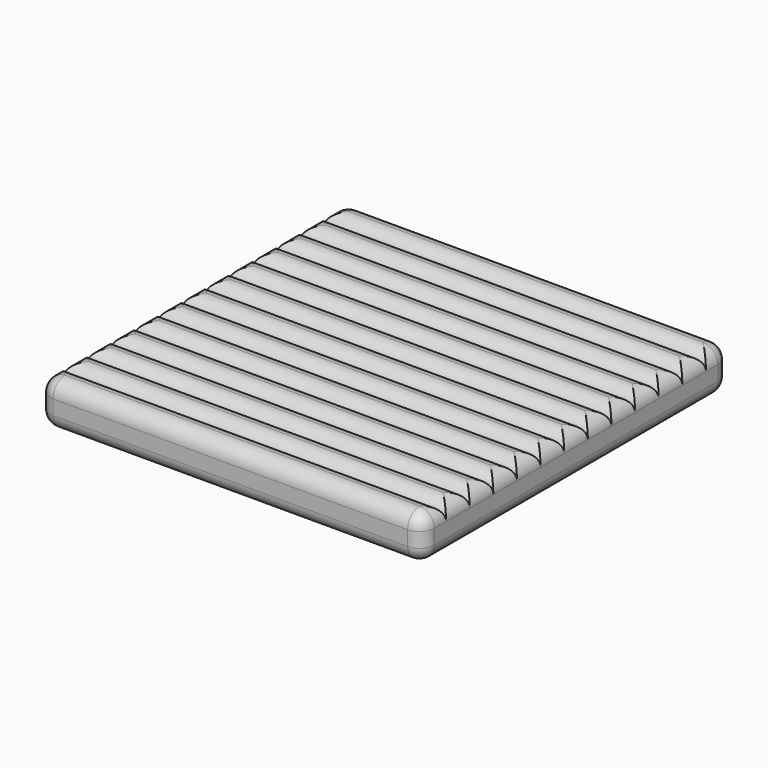
from build123d import *

# Parameters (mm, degrees)
F0_W         = 330.2
F0_H         = 330.2
F1_DEPTH     = 38.1
F2_R         = 12.7
F3_T1_DEPTH  = 12.7
F3_S5_W      = 12.7
F3_S5_H      = 12.7
F3_T6_DEPTH  = 12.7
F3_S11_W     = 12.7
F3_S11_H     = 12.7
F3_T12_DEPTH = 12.7
F3_S17_W     = 12.7
F3_S17_H     = 12.7
F3_T18_DEPTH = 12.7
F3_S23_W     = 12.7
F3_S23_H     = 12.7
F3_T24_DEPTH = 12.7
F3_S29_W     = 12.7
F3_S29_H     = 12.7
F3_T30_DEPTH = 12.7
F3_S35_W     = 12.7
F3_S35_H     = 12.7
F3_T36_DEPTH = 12.7
F3_S41_W     = 12.7
F3_S41_H     = 12.7
F3_T42_DEPTH = 12.7
F3_S47_W     = 12.7
F3_S47_H     = 12.7
F3_T48_DEPTH = 12.7
F5_DEPTH     = 330.201


# Not quite as in the source:
# - a fillet or chamfer that OpenCascade refuses, or shapes differently, is made with other operations: its cross-section is extruded or revolved along the edge and cut away or added
# - ends of sketch curves that miss each other by under 0.0002 mm in the source are joined


with BuildPart() as f1:
    # F0 (on Top) → F1 (new body)
    with BuildSketch(Plane.XY):
        with Locations((165.1, 165.1)):
            Rectangle(F0_W, F0_H)
    extrude(amount=F1_DEPTH)

    # F2
    f2_edges = [f1.edges().sort_by_distance(p)[0] for p in [
        (0, 165.1, 38.1),
        (165.1, 0, 38.1),
        (330.2, 165.1, 38.1),
        (165.1, 330.2, 38.1),
        (0, 165.1, 0),
        (165.1, 0, 0),
        (330.2, 165.1, 0),
        (165.1, 330.2, 0),
    ]]
    fillet(f2_edges, radius=F2_R)

    # F3: fillet of radius 12.7 on 4 edges, made by hand

    # F3_s2 → F3_t1 (cut)
    with BuildSketch(Plane.XY.offset(12.7)):
        with BuildLine():
            ThreePointArc((0, 12.7), (3.7197438789, 3.7197438789), (12.7, 0))
            Line((12.7, 0), (0, 0))
            Line((0, 0), (0, 12.7))
        make_face()
        with BuildLine():
            ThreePointArc((0, 317.5), (3.7197438789, 326.4802561211), (12.7, 330.2))
            Line((12.7, 330.2), (0, 330.2))
            Line((0, 330.2), (0, 317.5))
        make_face()
        with BuildLine():
            ThreePointArc((317.5, 330.2), (326.4802561211, 326.4802561211), (330.2, 317.5))
            Line((330.2, 317.5), (330.2, 330.2))
            Line((330.2, 330.2), (317.5, 330.2))
        make_face()
        with BuildLine():
            ThreePointArc((317.5, 0), (326.4802561211, 3.7197438789), (330.2, 12.7))
            Line((330.2, 12.7), (330.2, 0))
            Line((330.2, 0), (317.5, 0))
        make_face()
    extrude(amount=F3_T1_DEPTH, mode=Mode.SUBTRACT)


with BuildPart() as f3_tool4:
    # F3_s5 → F3_t6 (new body)
    with BuildSketch(Plane.XZ.offset(-12.7)):
        with Locations((323.85, 6.35)):
            Rectangle(F3_S5_W, F3_S5_H)
    extrude(amount=F3_T6_DEPTH)

    # F3_s7 → F3_t8 (revolve, cut)
    with BuildSketch(Plane(origin=(317.5, 12.7, 12.7), x_dir=(-0.7071067812, 0, 0.7071067812), z_dir=(0.7071067812, 0, 0.7071067812))):
        with BuildLine():
            ThreePointArc((0, -12.7), (12.7, 0), (0, 12.7))
            Line((0, 12.7), (0, -12.7))
        make_face()
    revolve(axis=Axis((317.5, 12.7, 12.7), (0, -1, 0)), mode=Mode.SUBTRACT)


with BuildPart() as f1_1:
    add(f1.part)

    # F3_t3: cut F3_tool4
    add(f3_tool4.part, mode=Mode.SUBTRACT)


with BuildPart() as f3_tool10:
    # F3_s11 → F3_t12 (new body)
    with BuildSketch(Plane.XZ.offset(-12.7)):
        with Locations((323.85, 31.75)):
            Rectangle(F3_S11_W, F3_S11_H)
    extrude(amount=F3_T12_DEPTH)

    # F3_s13 → F3_t14 (revolve, cut)
    with BuildSketch(Plane(origin=(317.5, 12.7, 25.4), x_dir=(-0.7071067812, 0, -0.7071067812), z_dir=(-0.7071067812, 0, 0.7071067812))):
        with BuildLine():
            ThreePointArc((0, -12.7), (12.7, 0), (0, 12.7))
            Line((0, 12.7), (0, -12.7))
        make_face()
    revolve(axis=Axis((317.5, 12.7, 25.4), (0, -1, 0)), mode=Mode.SUBTRACT)


with BuildPart() as f1_2:
    add(f1_1.part)

    # F3_t9: cut F3_tool10
    add(f3_tool10.part, mode=Mode.SUBTRACT)


with BuildPart() as f3_tool16:
    # F3_s17 → F3_t18 (new body)
    with BuildSketch(Plane.XZ.offset(-317.5)):
        with Locations((323.85, 6.35)):
            Rectangle(F3_S17_W, F3_S17_H)
    extrude(amount=-F3_T18_DEPTH)

    # F3_s19 → F3_t20 (revolve, cut)
    with BuildSketch(Plane(origin=(317.5, 317.5, 12.7), x_dir=(-0.7071067812, 0, 0.7071067812), z_dir=(-0.7071067812, 0, -0.7071067812))):
        with BuildLine():
            ThreePointArc((0, -12.7), (12.7, 0), (0, 12.7))
            Line((0, 12.7), (0, -12.7))
        make_face()
    revolve(axis=Axis((317.5, 317.5, 12.7), (0, 1, 0)), mode=Mode.SUBTRACT)


with BuildPart() as f1_3:
    add(f1_2.part)

    # F3_t15: cut F3_tool16
    add(f3_tool16.part, mode=Mode.SUBTRACT)


with BuildPart() as f3_tool22:
    # F3_s23 → F3_t24 (new body)
    with BuildSketch(Plane.XZ.offset(-317.5)):
        with Locations((323.85, 31.75)):
            Rectangle(F3_S23_W, F3_S23_H)
    extrude(amount=-F3_T24_DEPTH)

    # F3_s25 → F3_t26 (revolve, cut)
    with BuildSketch(Plane(origin=(317.5, 317.5, 25.4), x_dir=(-0.7071067812, 0, -0.7071067812), z_dir=(0.7071067812, 0, -0.7071067812))):
        with BuildLine():
            ThreePointArc((0, -12.7), (12.7, 0), (0, 12.7))
            Line((0, 12.7), (0, -12.7))
        make_face()
    revolve(axis=Axis((317.5, 317.5, 25.4), (0, 1, 0)), mode=Mode.SUBTRACT)


with BuildPart() as f1_4:
    add(f1_3.part)

    # F3_t21: cut F3_tool22
    add(f3_tool22.part, mode=Mode.SUBTRACT)


with BuildPart() as f3_tool28:
    # F3_s29 → F3_t30 (new body)
    with BuildSketch(Plane.YZ.offset(12.7)):
        with Locations((323.85, 6.35)):
            Rectangle(F3_S29_W, F3_S29_H)
    extrude(amount=-F3_T30_DEPTH)

    # F3_s31 → F3_t32 (revolve, cut)
    with BuildSketch(Plane(origin=(12.7, 317.5, 12.7), x_dir=(0, -0.7071067812, 0.7071067812), z_dir=(0, -0.7071067812, -0.7071067812))):
        with BuildLine():
            ThreePointArc((0, -12.7), (12.7, 0), (0, 12.7))
            Line((0, 12.7), (0, -12.7))
        make_face()
    revolve(axis=Axis((12.7, 317.5, 12.7), (-1, 0, 0)), mode=Mode.SUBTRACT)


with BuildPart() as f1_5:
    add(f1_4.part)

    # F3_t27: cut F3_tool28
    add(f3_tool28.part, mode=Mode.SUBTRACT)


with BuildPart() as f3_tool34:
    # F3_s35 → F3_t36 (new body)
    with BuildSketch(Plane.YZ.offset(12.7)):
        with Locations((323.85, 31.75)):
            Rectangle(F3_S35_W, F3_S35_H)
    extrude(amount=-F3_T36_DEPTH)

    # F3_s37 → F3_t38 (revolve, cut)
    with BuildSketch(Plane(origin=(12.7, 317.5, 25.4), x_dir=(0, -0.7071067812, -0.7071067812), z_dir=(0, 0.7071067812, -0.7071067812))):
        with BuildLine():
            ThreePointArc((0, -12.7), (12.7, 0), (0, 12.7))
            Line((0, 12.7), (0, -12.7))
        make_face()
    revolve(axis=Axis((12.7, 317.5, 25.4), (-1, 0, 0)), mode=Mode.SUBTRACT)


with BuildPart() as f1_6:
    add(f1_5.part)

    # F3_t33: cut F3_tool34
    add(f3_tool34.part, mode=Mode.SUBTRACT)


with BuildPart() as f3_tool40:
    # F3_s41 → F3_t42 (new body)
    with BuildSketch(Plane.YZ.offset(12.7)):
        with Locations((6.35, 6.35)):
            Rectangle(F3_S41_W, F3_S41_H)
    extrude(amount=-F3_T42_DEPTH)

    # F3_s43 → F3_t44 (revolve, cut)
    with BuildSketch(Plane(origin=(12.7, 12.7, 12.7), x_dir=(0, 0.7071067812, 0.7071067812), z_dir=(0, -0.7071067812, 0.7071067812))):
        with BuildLine():
            ThreePointArc((0, -12.7), (12.7, 0), (0, 12.7))
            Line((0, 12.7), (0, -12.7))
        make_face()
    revolve(axis=Axis((12.7, 12.7, 12.7), (-1, 0, 0)), mode=Mode.SUBTRACT)


with BuildPart() as f1_7:
    add(f1_6.part)

    # F3_t39: cut F3_tool40
    add(f3_tool40.part, mode=Mode.SUBTRACT)


with BuildPart() as f3_tool46:
    # F3_s47 → F3_t48 (new body)
    with BuildSketch(Plane.YZ.offset(12.7)):
        with Locations((6.35, 31.75)):
            Rectangle(F3_S47_W, F3_S47_H)
    extrude(amount=-F3_T48_DEPTH)

    # F3_s49 → F3_t50 (revolve, cut)
    with BuildSketch(Plane(origin=(12.7, 12.7, 25.4), x_dir=(0, 0.7071067812, -0.7071067812), z_dir=(0, 0.7071067812, 0.7071067812))):
        with BuildLine():
            ThreePointArc((0, -12.7), (12.7, 0), (0, 12.7))
            Line((0, 12.7), (0, -12.7))
        make_face()
    revolve(axis=Axis((12.7, 12.7, 25.4), (-1, 0, 0)), mode=Mode.SUBTRACT)


with BuildPart() as f1_8:
    add(f1_7.part)

    # F3_t45: cut F3_tool46
    add(f3_tool46.part, mode=Mode.SUBTRACT)

    # F4 (on face) → F5 (cut, through all)
    with BuildSketch(Plane.YZ.offset(330.2)):
        with BuildLine():
            Line((38.1, 38.1), (12.7, 38.1))
            ThreePointArc((12.7, 38.1), (21.6802561211, 34.3802561211), (25.4, 25.4))
            ThreePointArc((25.4, 25.4), (29.1197438789, 34.3802561211), (38.1, 38.1))
        make_face()
        with BuildLine():
            Line((317.5, 38.1), (292.0999955177, 38.1))
            ThreePointArc((292.0999955177, 38.1), (301.0802487413, 34.3802545363), (304.7999910355, 25.4))
            ThreePointArc((304.7999910355, 25.4), (308.5197380838, 34.3802592905), (317.5, 38.1))
        make_face()
        with BuildLine():
            Line((292.0999955177, 38.1), (266.7, 38.1))
            ThreePointArc((266.7, 38.1), (275.6802561211, 34.3802561211), (279.4, 25.4))
            ThreePointArc((279.4, 25.4), (283.1197364991, 34.3802577058), (292.0999955177, 38.1))
        make_face()
        with BuildLine():
            Line((266.7, 38.1), (241.3, 38.1))
            ThreePointArc((241.3, 38.1), (250.2802561211, 34.3802561211), (254, 25.4))
            ThreePointArc((254, 25.4), (257.7197438789, 34.3802561211), (266.7, 38.1))
        make_face()
        with BuildLine():
            Line((241.3, 38.1), (215.9, 38.1))
            ThreePointArc((215.9, 38.1), (224.8802561211, 34.3802561211), (228.6, 25.4))
            ThreePointArc((228.6, 25.4), (232.3197438789, 34.3802561211), (241.3, 38.1))
        make_face()
        with BuildLine():
            Line((215.9, 38.1), (190.5, 38.1))
            ThreePointArc((190.5, 38.1), (199.4802561211, 34.3802561211), (203.2, 25.4))
            ThreePointArc((203.2, 25.4), (206.9197438789, 34.3802561211), (215.9, 38.1))
        make_face()
        with BuildLine():
            Line((190.5, 38.1), (165.1, 38.1))
            ThreePointArc((165.1, 38.1), (174.0802561211, 34.3802561211), (177.8, 25.4))
            ThreePointArc((177.8, 25.4), (181.5197438789, 34.3802561211), (190.5, 38.1))
        make_face()
        with BuildLine():
            Line((165.1, 38.1), (139.7, 38.1))
            ThreePointArc((139.7, 38.1), (148.6802561211, 34.3802561211), (152.4, 25.4))
            ThreePointArc((152.4, 25.4), (156.1197438789, 34.3802561211), (165.1, 38.1))
        make_face()
        with BuildLine():
            Line((139.7, 38.1), (114.3, 38.1))
            ThreePointArc((114.3, 38.1), (123.2802561211, 34.3802561211), (127, 25.4))
            ThreePointArc((127, 25.4), (130.7197438789, 34.3802561211), (139.7, 38.1))
        make_face()
        with BuildLine():
            Line((114.3, 38.1), (88.9, 38.1))
            ThreePointArc((88.9, 38.1), (97.8802561211, 34.3802561211), (101.6, 25.4))
            ThreePointArc((101.6, 25.4), (105.3197438789, 34.3802561211), (114.3, 38.1))
        make_face()
        with BuildLine():
            Line((88.9, 38.1), (63.5, 38.1))
            ThreePointArc((63.5, 38.1), (72.4802561211, 34.3802561211), (76.2, 25.4))
            ThreePointArc((76.2, 25.4), (79.9197438789, 34.3802561211), (88.9, 38.1))
        make_face()
        with BuildLine():
            Line((63.5, 38.1), (38.1, 38.1))
            ThreePointArc((38.1, 38.1), (47.0802561211, 34.3802561211), (50.8, 25.4))
            ThreePointArc((50.8, 25.4), (54.5197438789, 34.3802561211), (63.5, 38.1))
        make_face()
    extrude(amount=-F5_DEPTH, mode=Mode.SUBTRACT)


solid = f1_8.part
